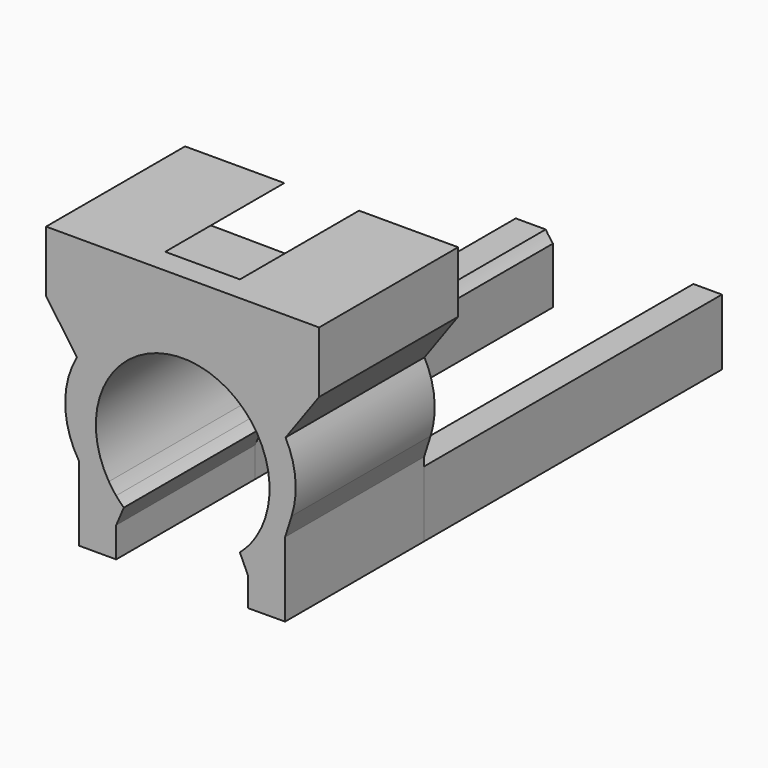
from build123d import *

# Parameters (mm, degrees)
F1_DEPTH = 7
F2_DEPTH = 6
F3_DEPTH = 15


# Not quite as in the source:
# - a feature names something its author has since deleted; it is built from what else it names


with BuildPart() as f1:
    # F0 (on Front) → F1 (new body)
    with BuildSketch(Plane.XZ):
        with BuildLine():
            Line((-4.090710345, -1.9507641112), (-3.3236176952, -1.6008211246))
            Line((-3.3236176952, -1.6008211246), (-3.3236176952, -2.2903047641))
            Line((-3.3236176952, -2.2903047641), (-2.8842022451, -2.2903047641))
            ThreePointArc((-2.8842022451, -2.2903047641), (0.0905031972, 3.0539098469), (3.0652086395, -2.2903047641))
            Line((3.0652086395, -2.2903047641), (3.4491920394, -2.2903047641))
            Line((3.4491920394, -2.2903047641), (3.4491920394, -1.6408955531))
            Line((3.4491920394, -1.6408955531), (4.2162846892, -1.9507641112))
            Line((4.2162846892, -1.9507641112), (4.4794066601, -1.1210844752))
            ThreePointArc((4.4794066601, -1.1210844752), (4.6290079186, 0.2570213688), (4.2328723206, 1.5854162054))
            Line((4.2328723206, 1.5854162054), (5.5865912817, 3.465253188))
            Line((5.5865912817, 3.465253188), (5.5865912817, 5.931237081))
            Line((5.5865912817, 5.931237081), (1.5955031972, 5.931237081))
            Line((1.5955031972, 5.931237081), (4.5903746292, 3.397220974))
            Line((4.5903746292, 3.397220974), (0.0905031972, 3.431237081))
            Line((0.0905031972, 3.431237081), (-4.4093682348, 3.465253188))
            Line((-4.4093682348, 3.465253188), (-1.4144968028, 5.931237081))
            Line((-1.4144968028, 5.931237081), (-5.4144968028, 5.931237081))
            Line((-5.4144968028, 5.931237081), (-5.4144968028, 3.465253188))
            Line((-5.4144968028, 3.465253188), (-4.1709532845, 1.6969049432))
            ThreePointArc((-4.1709532845, 1.6969049432), (-4.6426172218, -0.138188052), (-4.090710345, -1.9507641112))
        make_face()
        Polygon((-3.3236176952, -2.2903047641), (-3.3236176952, -1.6008211246), (-4.090710345, -1.9507641112), (-4.090710345, -2.2903047641), align=None)
        with BuildLine():
            Line((-2.8842022451, -2.2903047641), (-3.3236176952, -2.2903047641))
            Line((-3.3236176952, -2.2903047641), (-4.090710345, -2.2903047641))
            Line((-4.090710345, -2.2903047641), (-4.090710345, -4.9565606735))
            Line((-4.090710345, -4.9565606735), (-3.3236176952, -4.9565606735))
            Line((-3.3236176952, -4.9565606735), (-2.590710345, -4.9565606735))
            Line((-2.590710345, -4.9565606735), (-2.590710345, -3.7436034497))
            Line((-2.590710345, -3.7436034497), (-2.590710345, -2.6957776739))
            ThreePointArc((-2.590710345, -2.6957776739), (-2.7447140714, -2.4982945873), (-2.8842022451, -2.2903047641))
        make_face()
        with BuildLine():
            Line((3.4491920394, -2.2903047641), (3.0652086395, -2.2903047641))
            ThreePointArc((3.0652086395, -2.2903047641), (2.9005872431, -2.5325770701), (2.7162846892, -2.76023612))
            Line((2.7162846892, -2.76023612), (2.7162846892, -3.7879117456))
            Line((2.7162846892, -3.7879117456), (2.7162846892, -4.9565606735))
            Line((2.7162846892, -4.9565606735), (4.2162846892, -4.9497258588))
            Line((4.2162846892, -4.9497258588), (4.2162846892, -2.2903047641))
            Line((4.2162846892, -2.2903047641), (3.4491920394, -2.2903047641))
        make_face()
        with BuildLine():
            ThreePointArc((-2.2823536237, -3.0189388676), (-2.4416925097, -2.8622823851), (-2.590710345, -2.6957776739))
            Line((-2.590710345, -2.6957776739), (-2.590710345, -3.7436034497))
            Line((-2.590710345, -3.7436034497), (-2.2823536237, -3.0189388676))
        make_face()
        Polygon((3.4491920394, -1.6408955531), (3.4491920394, -2.2903047641), (4.2162846892, -2.2903047641), (4.2162846892, -1.9507641112), align=None)
        with BuildLine():
            Line((2.7162846892, -3.7879117456), (2.7162846892, -2.76023612))
            ThreePointArc((2.7162846892, -2.76023612), (2.5594926434, -2.9268342178), (2.39215173, -3.0828332258))
            Line((2.39215173, -3.0828332258), (2.7162846892, -3.7879117456))
        make_face()
        Polygon((1.5955031972, 5.931237081), (-1.4144968028, 5.931237081), (-4.4093682348, 3.465253188), (0.0905031972, 3.431237081), (4.5903746292, 3.397220974), align=None)
    extrude(amount=F1_DEPTH)

    # F0 (on Front) → F2 (cut)
    with BuildSketch(Plane.XZ):
        Polygon((1.5955031972, 5.931237081), (-1.4144968028, 5.931237081), (-4.4093682348, 3.465253188), (0.0905031972, 3.431237081), (4.5903746292, 3.397220974), align=None)
    extrude(amount=F2_DEPTH, mode=Mode.SUBTRACT)

    # F0 (on Front) → F3 (join)
    with BuildSketch(Plane.XZ):
        with BuildLine():
            Line((-2.8842022451, -2.2903047641), (-3.3236176952, -2.2903047641))
            Line((-3.3236176952, -2.2903047641), (-4.090710345, -2.2903047641))
            Line((-4.090710345, -2.2903047641), (-4.090710345, -4.9565606735))
            Line((-4.090710345, -4.9565606735), (-3.3236176952, -4.9565606735))
            Line((-3.3236176952, -4.9565606735), (-2.590710345, -4.9565606735))
            Line((-2.590710345, -4.9565606735), (-2.590710345, -3.7436034497))
            Line((-2.590710345, -3.7436034497), (-2.590710345, -2.6957776739))
            ThreePointArc((-2.590710345, -2.6957776739), (-2.7447140714, -2.4982945873), (-2.8842022451, -2.2903047641))
        make_face()
        with BuildLine():
            Line((3.4491920394, -2.2903047641), (3.0652086395, -2.2903047641))
            ThreePointArc((3.0652086395, -2.2903047641), (2.9005872431, -2.5325770701), (2.7162846892, -2.76023612))
            Line((2.7162846892, -2.76023612), (2.7162846892, -3.7879117456))
            Line((2.7162846892, -3.7879117456), (2.7162846892, -4.9565606735))
            Line((2.7162846892, -4.9565606735), (4.2162846892, -4.9497258588))
            Line((4.2162846892, -4.9497258588), (4.2162846892, -2.2903047641))
            Line((4.2162846892, -2.2903047641), (3.4491920394, -2.2903047641))
        make_face()
    extrude(amount=-F3_DEPTH)


solid = f1.part
